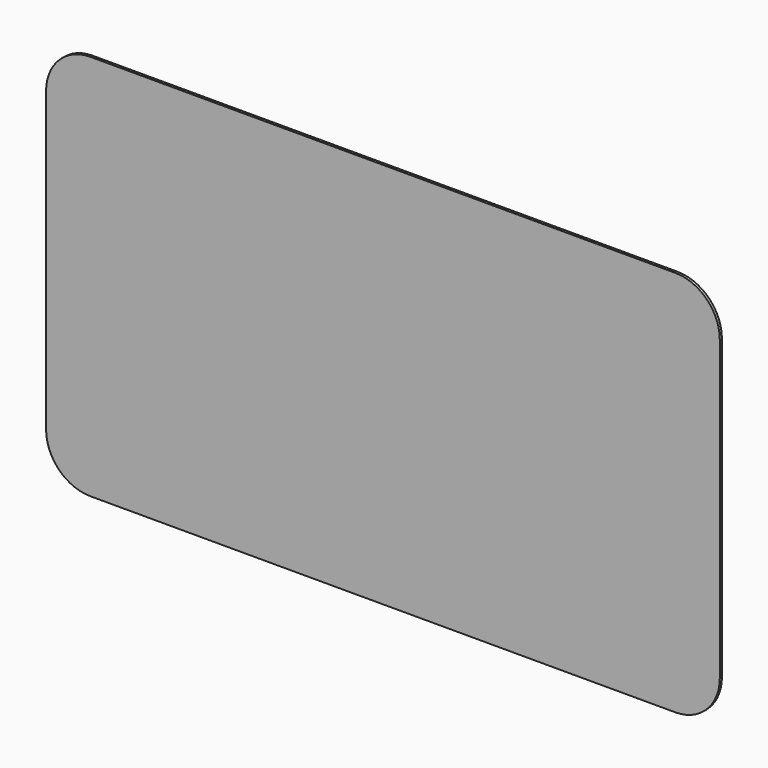
from build123d import *

# Parameters (mm, degrees)
F1_DEPTH   = 0.762
F2_W       = 166.2938
F2_H       = 100.7999
F3_DEPTH   = 5.08
F4_W       = 14.478
F4_H       = 7.874
F4_R       = 1.27
F4_W_2     = 7.874
F4_H_2     = 14.478
F5_DEPTH   = 2.413
F6_SIZE2   = 3.80999
F6_SIZE    = 2.41299
F6_2_SIZE2 = 3.80999
F6_2_SIZE  = 2.41299
F6_3_SIZE2 = 3.80999
F6_3_SIZE  = 2.41299
F6_4_SIZE2 = 3.80999
F6_4_SIZE  = 2.41299
F6_5_SIZE2 = 3.80999
F6_5_SIZE  = 2.41299
F6_6_SIZE2 = 3.80999
F6_6_SIZE  = 2.41299
F6_7_SIZE2 = 3.80999
F6_7_SIZE  = 2.41299
F6_8_SIZE2 = 3.80999
F6_8_SIZE  = 2.41299
F6_9_SIZE2 = 3.80999
F6_9_SIZE  = 2.41299
F7_SIZE2   = 3.80999
F7_SIZE    = 2.41299
F7_2_SIZE2 = 3.80999
F7_2_SIZE  = 2.41299
F7_3_SIZE2 = 3.80999
F7_3_SIZE  = 2.41299
F7_4_SIZE2 = 3.80999
F7_4_SIZE  = 2.41299
F7_5_SIZE2 = 3.80999
F7_5_SIZE  = 2.41299
F7_6_SIZE2 = 3.80999
F7_6_SIZE  = 2.41299
F7_7_SIZE2 = 3.80999
F7_7_SIZE  = 2.41299
F9_DEPTH   = 73.533
F11_DEPTH  = 64.2493
F12_W      = 40.005
F12_H      = 5.08
F13_DEPTH  = 3.34264


# Not quite as in the source:
# - a fillet or chamfer is up to 0.001 mm smaller than in the source, because OpenCascade refuses the exact size


with BuildPart() as f1:
    # F0 (on Front) → F1 (new body)
    with BuildSketch(Plane.XZ):
        with BuildLine():
            ThreePointArc((96.43872, 42.67327), (92.7189761211, 51.6535261211), (83.73872, 55.37327))
            Line((83.73872, 55.37327), (-83.73872, 55.37327))
            ThreePointArc((-83.73872, 55.37327), (-92.7189761211, 51.6535261211), (-96.43872, 42.67327))
            Line((-96.43872, 42.67327), (-96.43872, -42.67327))
            ThreePointArc((-96.43872, -42.67327), (-92.7189761211, -51.6535261211), (-83.73872, -55.37327))
            Line((-83.73872, -55.37327), (83.73872, -55.37327))
            ThreePointArc((83.73872, -55.37327), (92.7189761211, -51.6535261211), (96.43872, -42.67327))
            Line((96.43872, -42.67327), (96.43872, 42.67327))
        make_face()
    extrude(amount=F1_DEPTH)

    # F2 (on face) → F3 (join)
    with BuildSketch(Plane(origin=(0, 0, 0), x_dir=(-1, 0, 0), z_dir=(0, 1, 0))):
        with Locations((-1.60782, -1.63068)):
            Rectangle(F2_W, F2_H)
    extrude(amount=F3_DEPTH)

    # F4 (on face) → F5 (join)
    with BuildSketch(Plane(origin=(0, 5.08, 0), x_dir=(-1, 0, 0), z_dir=(0, 1, 0))):
        with Locations((-63.98768, 33.78327)):
            Rectangle(F4_W, F4_H)
        with Locations((-63.98768, 33.78327)):
            Circle(F4_R, mode=Mode.SUBTRACT)
        with Locations((-63.98768, -31.87573)):
            Rectangle(F4_W, F4_H)
        with Locations((-63.98768, -31.87573)):
            Circle(F4_R, mode=Mode.SUBTRACT)
        with Locations((62.22492, 33.78327)):
            Rectangle(F4_W, F4_H)
        with Locations((62.22492, 33.78327)):
            Circle(F4_R, mode=Mode.SUBTRACT)
        with Locations((62.22492, -31.87573)):
            Rectangle(F4_W, F4_H)
        with Locations((62.22492, -31.87573)):
            Circle(F4_R, mode=Mode.SUBTRACT)
        with Locations((-37.26942, 28.95473)):
            Rectangle(F4_W_2, F4_H_2)
        with Locations((-37.26942, 28.95473)):
            Circle(F4_R, mode=Mode.SUBTRACT)
        with Locations((19.10588, 28.95473)):
            Rectangle(F4_W_2, F4_H_2)
        with Locations((19.10588, 28.95473)):
            Circle(F4_R, mode=Mode.SUBTRACT)
        with Locations((-37.26942, -19.30527)):
            Rectangle(F4_W_2, F4_H_2)
        with Locations((-37.26942, -19.30527)):
            Circle(F4_R, mode=Mode.SUBTRACT)
        with Locations((19.10588, -19.30527)):
            Rectangle(F4_W_2, F4_H_2)
        with Locations((19.10588, -19.30527)):
            Circle(F4_R, mode=Mode.SUBTRACT)
    extrude(amount=F5_DEPTH)

    # F6 (size 2.413 and 3.81 in the source; OpenCascade refuses exactly that, so slightly less here)
    f6_edges = [f1.edges().sort_by_distance(p)[0] for p in [
        (56.74868, 7.493, 33.78327),
    ]]
    f6_side = f1.faces().sort_by_distance((56.74868, 6.2865, 33.78327))[0]
    chamfer(f6_edges, length=F6_SIZE, length2=F6_SIZE2, reference=f6_side)

    # F6#2 (size 2.413 and 3.81 in the source; OpenCascade refuses exactly that, so slightly less here)
    f6_2_edges = [f1.edges().sort_by_distance(p)[0] for p in [
        (71.22668, 7.493, 33.78327),
    ]]
    f6_2_side = f1.faces().sort_by_distance((71.22668, 6.2865, 33.78327))[0]
    chamfer(f6_2_edges, length=F6_2_SIZE, length2=F6_2_SIZE2, reference=f6_2_side)

    # F6#3 (size 2.413 and 3.81 in the source; OpenCascade refuses exactly that, so slightly less here)
    f6_3_edges = [f1.edges().sort_by_distance(p)[0] for p in [
        (56.74868, 7.493, -31.87573),
    ]]
    f6_3_side = f1.faces().sort_by_distance((56.74868, 6.2865, -31.87573))[0]
    chamfer(f6_3_edges, length=F6_3_SIZE, length2=F6_3_SIZE2, reference=f6_3_side)

    # F6#4 (size 2.413 and 3.81 in the source; OpenCascade refuses exactly that, so slightly less here)
    f6_4_edges = [f1.edges().sort_by_distance(p)[0] for p in [
        (37.26942, 7.493, -26.54427),
    ]]
    f6_4_side = f1.faces().sort_by_distance((37.26942, 6.2865, -26.54427))[0]
    chamfer(f6_4_edges, length=F6_4_SIZE, length2=F6_4_SIZE2, reference=f6_4_side)

    # F6#5 (size 2.413 and 3.81 in the source; OpenCascade refuses exactly that, so slightly less here)
    f6_5_edges = [f1.edges().sort_by_distance(p)[0] for p in [
        (37.26942, 7.493, 21.71573),
    ]]
    f6_5_side = f1.faces().sort_by_distance((37.26942, 6.2865, 21.71573))[0]
    chamfer(f6_5_edges, length=F6_5_SIZE, length2=F6_5_SIZE2, reference=f6_5_side)

    # F6#6 (size 2.413 and 3.81 in the source; OpenCascade refuses exactly that, so slightly less here)
    f6_6_edges = [f1.edges().sort_by_distance(p)[0] for p in [
        (-19.10588, 7.493, -26.54427),
    ]]
    f6_6_side = f1.faces().sort_by_distance((-19.10588, 6.2865, -26.54427))[0]
    chamfer(f6_6_edges, length=F6_6_SIZE, length2=F6_6_SIZE2, reference=f6_6_side)

    # F6#7 (size 2.413 and 3.81 in the source; OpenCascade refuses exactly that, so slightly less here)
    f6_7_edges = [f1.edges().sort_by_distance(p)[0] for p in [
        (-19.10588, 7.493, 21.71573),
    ]]
    f6_7_side = f1.faces().sort_by_distance((-19.10588, 6.2865, 21.71573))[0]
    chamfer(f6_7_edges, length=F6_7_SIZE, length2=F6_7_SIZE2, reference=f6_7_side)

    # F6#8 (size 2.413 and 3.81 in the source; OpenCascade refuses exactly that, so slightly less here)
    f6_8_edges = [f1.edges().sort_by_distance(p)[0] for p in [
        (-69.46392, 7.493, 33.78327),
    ]]
    f6_8_side = f1.faces().sort_by_distance((-69.46392, 6.2865, 33.78327))[0]
    chamfer(f6_8_edges, length=F6_8_SIZE, length2=F6_8_SIZE2, reference=f6_8_side)

    # F6#9 (size 2.413 and 3.81 in the source; OpenCascade refuses exactly that, so slightly less here)
    f6_9_edges = [f1.edges().sort_by_distance(p)[0] for p in [
        (-69.46392, 7.493, -31.87573),
    ]]
    f6_9_side = f1.faces().sort_by_distance((-69.46392, 6.2865, -31.87573))[0]
    chamfer(f6_9_edges, length=F6_9_SIZE, length2=F6_9_SIZE2, reference=f6_9_side)

    # F7 (size 2.413 and 3.81 in the source; OpenCascade refuses exactly that, so slightly less here)
    f7_edges = [f1.edges().sort_by_distance(p)[0] for p in [
        (37.26942, 7.493, 36.19373),
    ]]
    f7_side = f1.faces().sort_by_distance((37.26942, 6.2865, 36.19373))[0]
    chamfer(f7_edges, length=F7_SIZE, length2=F7_SIZE2, reference=f7_side)

    # F7#2 (size 2.413 and 3.81 in the source; OpenCascade refuses exactly that, so slightly less here)
    f7_2_edges = [f1.edges().sort_by_distance(p)[0] for p in [
        (71.22668, 7.493, -31.87573),
    ]]
    f7_2_side = f1.faces().sort_by_distance((71.22668, 6.2865, -31.87573))[0]
    chamfer(f7_2_edges, length=F7_2_SIZE, length2=F7_2_SIZE2, reference=f7_2_side)

    # F7#3 (size 2.413 and 3.81 in the source; OpenCascade refuses exactly that, so slightly less here)
    f7_3_edges = [f1.edges().sort_by_distance(p)[0] for p in [
        (37.26942, 7.493, -12.06627),
    ]]
    f7_3_side = f1.faces().sort_by_distance((37.26942, 6.2865, -12.06627))[0]
    chamfer(f7_3_edges, length=F7_3_SIZE, length2=F7_3_SIZE2, reference=f7_3_side)

    # F7#4 (size 2.413 and 3.81 in the source; OpenCascade refuses exactly that, so slightly less here)
    f7_4_edges = [f1.edges().sort_by_distance(p)[0] for p in [
        (-19.10588, 7.493, -12.06627),
    ]]
    f7_4_side = f1.faces().sort_by_distance((-19.10588, 6.2865, -12.06627))[0]
    chamfer(f7_4_edges, length=F7_4_SIZE, length2=F7_4_SIZE2, reference=f7_4_side)

    # F7#5 (size 2.413 and 3.81 in the source; OpenCascade refuses exactly that, so slightly less here)
    f7_5_edges = [f1.edges().sort_by_distance(p)[0] for p in [
        (-19.10588, 7.493, 36.19373),
    ]]
    f7_5_side = f1.faces().sort_by_distance((-19.10588, 6.2865, 36.19373))[0]
    chamfer(f7_5_edges, length=F7_5_SIZE, length2=F7_5_SIZE2, reference=f7_5_side)

    # F7#6 (size 2.413 and 3.81 in the source; OpenCascade refuses exactly that, so slightly less here)
    f7_6_edges = [f1.edges().sort_by_distance(p)[0] for p in [
        (-54.98592, 7.493, 33.78327),
    ]]
    f7_6_side = f1.faces().sort_by_distance((-54.98592, 6.2865, 33.78327))[0]
    chamfer(f7_6_edges, length=F7_6_SIZE, length2=F7_6_SIZE2, reference=f7_6_side)

    # F7#7 (size 2.413 and 3.81 in the source; OpenCascade refuses exactly that, so slightly less here)
    f7_7_edges = [f1.edges().sort_by_distance(p)[0] for p in [
        (-54.98592, 7.493, -31.87573),
    ]]
    f7_7_side = f1.faces().sort_by_distance((-54.98592, 6.2865, -31.87573))[0]
    chamfer(f7_7_edges, length=F7_7_SIZE, length2=F7_7_SIZE2, reference=f7_7_side)

    # F8 (on face) → F9 (cut, through all)
    with BuildSketch(Plane.XY.offset(37.72027)):
        Polygon((-65.5802524895, 7.239), (-68.9891998579, 5.08), (-55.4606401421, 5.08), (-58.8695875105, 7.239), align=None)
        Polygon((60.6323475105, 7.239), (57.2234001421, 5.08), (70.7519598579, 5.08), (67.3430124895, 7.239), align=None)
    extrude(amount=-F9_DEPTH, mode=Mode.SUBTRACT)

    # F10 (on face) → F11 (cut, through all)
    with BuildSketch(Plane(origin=(-23.04288, 0, 0), x_dir=(0, -1, 0), z_dir=(-1, 0, 0))):
        Polygon((-7.239, -22.6606024895), (-5.08, -26.0695498579), (-5.08, -12.5409901421), (-7.239, -15.9499375105), align=None)
        Polygon((-7.239, 25.5993975105), (-5.08, 22.1904501421), (-5.08, 35.7190098579), (-7.239, 32.3100624895), align=None)
    extrude(amount=-F11_DEPTH, mode=Mode.SUBTRACT)

    # F12 (on face) → F13 (join, through all)
    with BuildSketch(Plane(origin=(0, 0, -52.03063), x_dir=(1, 0, 0), z_dir=(0, 0, -1))):
        with Locations((-0.06858, -2.54)):
            Rectangle(F12_W, F12_H)
    extrude(amount=F13_DEPTH)


solid = f1.part
